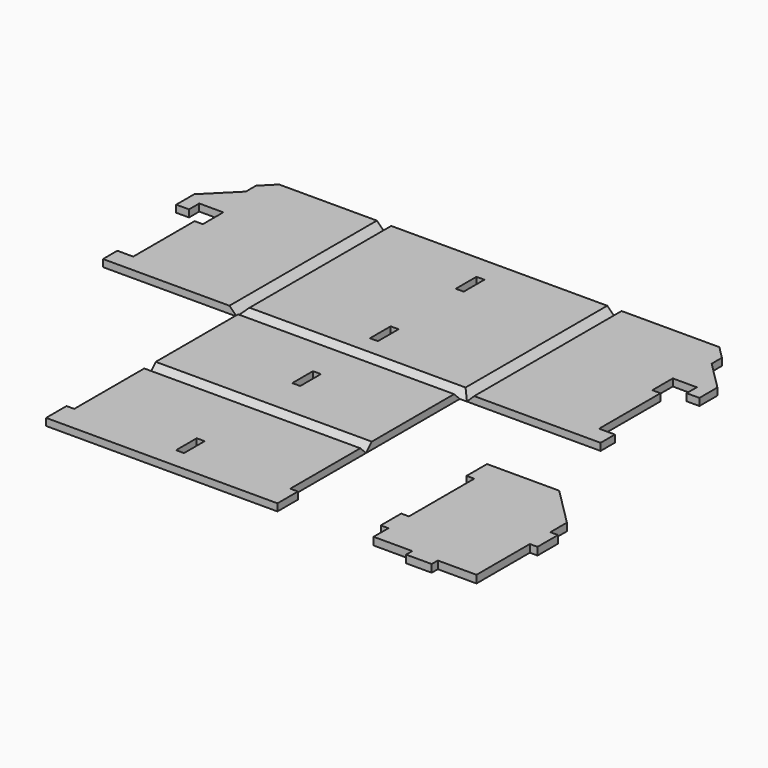
from build123d import *

# Parameters (mm, degrees)
F1_DEPTH   = 2.8
F2_SIZE    = 2.79999
F2_2_SIZE  = 2.79999
F3_DEPTH   = 2.8
F4_SIZE    = 2.79999
F5_W       = 3.1
F5_H       = 10.1
F6_DEPTH   = 3
F0_W       = 84.4
F0_H       = 45.8
F7_DEPTH   = 2.8
F8_SIZE    = 2.79999
F0_H_2     = 47
F9_DEPTH   = 2.8
F10_SIZE   = 2.79999
F11_W      = 10
F11_H      = 2.8
F12_DEPTH  = 3
F15_W      = 3.1
F15_H      = 10.1
F14_W      = 3.1
F14_H      = 10.1
F16_DEPTH  = 4
F18_DEPTH  = 3
F19_SIZE   = 5
F19_2_SIZE = 5
F20_SIZE   = 15


# Not quite as in the source:
# - a fillet or chamfer is up to 0.001 mm smaller than in the source, because OpenCascade refuses the exact size


with BuildPart() as f1:
    # F0 (on Top) → F1 (new body)
    with BuildSketch(Plane.XY):
        Polygon((-45, -36), (-45, 36), (-91, 36), (-91, 26), (-102.2, 14.8), (-102.2, 6), (-97.2, 6), (-97.2, 11), (-91, 11), (-87.8, 11), (-87.8, 1), (-91, 1), (-91, -29), (-97.2, -29), (-97.2, -36), (-91, -36), align=None)
    extrude(amount=F1_DEPTH)

    # F2 (size 2.8 in the source; OpenCascade refuses exactly that, so slightly less here)
    f2_edges = [f1.edges().sort_by_distance(p)[0] for p in [
        (-45, 0, 2.8),
    ]]
    chamfer(f2_edges, length=F2_SIZE)

    # F19
    f19_edges = [f1.edges().sort_by_distance(p)[0] for p in [
        (-91, 36, 1.4),
    ]]
    chamfer(f19_edges, length=F19_SIZE)


with BuildPart() as f1b:
    # F0 (on Top) → F1, piece 2 (new body)
    with BuildSketch(Plane.XY):
        Polygon((45, 36), (45, -36), (91, -36), (97.2, -36), (97.2, -29), (91, -29), (91, 1), (87.8, 1), (87.8, 11), (91, 11), (97.2, 11), (97.2, 6), (102.2, 6), (102.2, 14.8), (91, 26), (91, 36), align=None)
    extrude(amount=F1_DEPTH)

    # F2#2 (size 2.8 in the source; OpenCascade refuses exactly that, so slightly less here)
    f2_2_edges = [f1b.edges().sort_by_distance(p)[0] for p in [
        (45, 0, 2.8),
    ]]
    chamfer(f2_2_edges, length=F2_2_SIZE)

    # F19#2
    f19_2_edges = [f1b.edges().sort_by_distance(p)[0] for p in [
        (91, 36, 1.4),
    ]]
    chamfer(f19_2_edges, length=F19_2_SIZE)


with BuildPart() as f3:
    # F0 (on Top) → F3 (new body)
    with BuildSketch(Plane.XY):
        Polygon((42.2, -36), (45, -36), (45, 36), (-45, 36), (-45, -36), (-42.2, -36), align=None)
    extrude(amount=F3_DEPTH)

    # F4 (size 2.8 in the source; OpenCascade refuses exactly that, so slightly less here)
    f4_edges = [f3.edges().sort_by_distance(p)[0] for p in [
        (45, 0, 2.8),
        (-45, 0, 2.8),
        (0, -36, 2.8),
    ]]
    chamfer(f4_edges, length=F4_SIZE)

    # F5 (on face) → F6 (cut)
    with BuildSketch(Plane.XY.offset(2.8)):
        with Locations((0.65, 20.95)):
            Rectangle(F5_W, F5_H)
        with Locations((0.65, -20.95)):
            Rectangle(F5_W, F5_H)
    extrude(amount=-F6_DEPTH, mode=Mode.SUBTRACT)


with BuildPart() as f7:
    # F0 (on Top) → F7 (new body)
    with BuildSketch(Plane.XY):
        with Locations((0, -58.9)):
            Rectangle(F0_W, F0_H)
    extrude(amount=F7_DEPTH)

    # F8 (size 2.8 in the source; OpenCascade refuses exactly that, so slightly less here)
    f8_edges = [f7.edges().sort_by_distance(p)[0] for p in [
        (0, -36, 2.8),
        (0, -81.8, 2.8),
    ]]
    chamfer(f8_edges, length=F8_SIZE)


with BuildPart() as f9:
    # F0 (on Top) → F9 (new body)
    with BuildSketch(Plane.XY):
        with Locations((0, -105.3)):
            Rectangle(F0_W, F0_H_2)
    extrude(amount=F9_DEPTH)

    # F10 (size 2.8 in the source; OpenCascade refuses exactly that, so slightly less here)
    f10_edges = [f9.edges().sort_by_distance(p)[0] for p in [
        (0, -81.8, 2.8),
    ]]
    chamfer(f10_edges, length=F10_SIZE)

    # F11 (on face) → F12 (join)
    with BuildSketch(Plane(origin=(-42.2, 0, 0), x_dir=(0, -1, 0), z_dir=(-1, 0, 0))):
        with Locations((123.8, 1.4)):
            Rectangle(F11_W, F11_H)
    extrude(amount=F12_DEPTH)

    # F13: F9 across plane


with BuildPart() as f9_1:
    add(f9.part)
    add(f9.part.mirror(Plane.YZ))


with BuildPart() as f16_tool:
    # F15 (on face) + F14 (on face) → F16 (new body)
    with BuildSketch(Plane.XY.offset(2.8)):
        with Locations((0.65, -115.65)):
            Rectangle(F15_W, F15_H)
    with BuildSketch(Plane.XY.offset(2.8)):
        with Locations((0.65, -58.9)):
            Rectangle(F14_W, F14_H)
    extrude(amount=-F16_DEPTH)


with BuildPart() as f7_1:
    add(f7.part)

    # F16: cut by f16_tool
    add(f16_tool.part, mode=Mode.SUBTRACT)


with BuildPart() as f9_2:
    add(f9_1.part)

    # F16: cut by f16_tool
    add(f16_tool.part, mode=Mode.SUBTRACT)


with BuildPart() as f18:
    # F17 (on Top) → F18 (new body)
    with BuildSketch(Plane.XY):
        Polygon((122.3451334953, -68.8853332162), (82.1451334953, -68.8853332162), (79.1451334953, -68.8853332162), (79.1451334953, -78.8853332162), (82.1451334953, -78.8853332162), (82.1451334953, -110.7853332162), (79.1451334953, -110.7853332162), (79.1451334953, -120.7853332162), (82.1451334953, -120.7853332162), (82.1451334953, -128.0353332162), (97.2451334953, -128.0353332162), (97.2451334953, -131.0353332162), (102.2451334953, -131.0353332162), (107.2451334953, -131.0353332162), (107.2451334953, -128.0353332162), (122.3451334953, -128.0353332162), (122.3451334953, -101.9853332162), (125.3451334953, -101.9853332162), (125.3451334953, -91.9853332162), (122.3451334953, -91.9853332162), align=None)
    extrude(amount=F18_DEPTH)

    # F20
    f20_edges = [f18.edges().sort_by_distance(p)[0] for p in [
        (122.345133, -68.885333, 1.5),
    ]]
    chamfer(f20_edges, length=F20_SIZE)


solid = Compound([f1.part, f1b.part, f3.part, f7_1.part, f9_2.part, f18.part])
